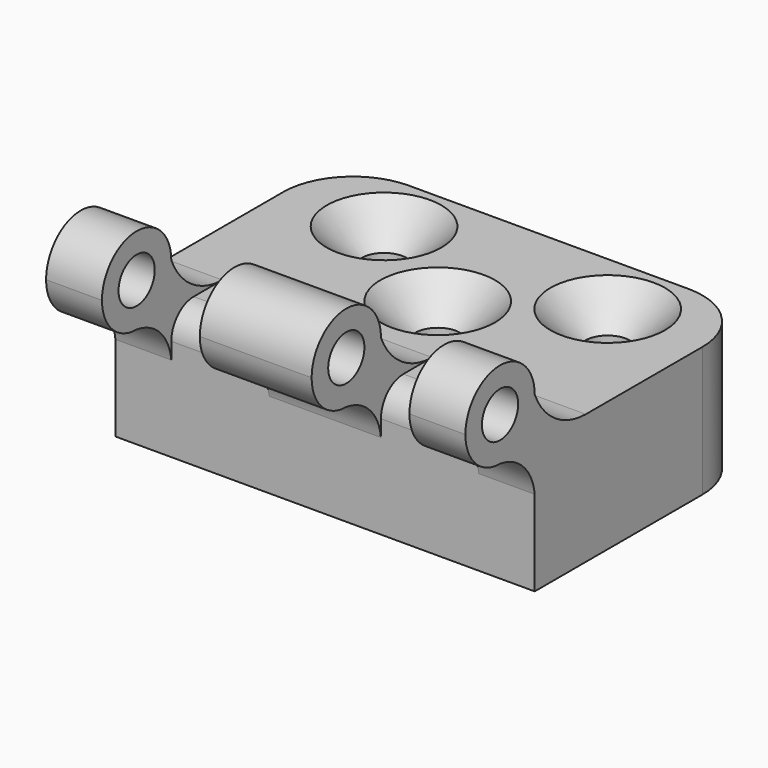
from build123d import *

# Parameters (mm, degrees)
F0_W      = 30
F0_H      = 20
F0_R      = 1.6
F1_DEPTH  = 5
F3_DEPTH  = 30
F7_DEPTH  = 7
F9_DEPTH  = 7
F10_SIZE  = 2.5
F11_R     = 5
F12_R     = 1.6200998357
F13_DEPTH = 30.001
F14_R     = 2
F15_DEPTH = 4.3


with BuildPart() as f1:
    # F0 (on Top) → F1 (new body)
    with BuildSketch(Plane.XY):
        Rectangle(F0_W, F0_H)
        with Locations((-8, 5.2767994255)):
            Circle(F0_R, mode=Mode.SUBTRACT)
        with Locations((0, 0.0767994255)):
            Circle(F0_R, mode=Mode.SUBTRACT)
        with Locations((8, 5.2767994255)):
            Circle(F0_R, mode=Mode.SUBTRACT)
    extrude(amount=F1_DEPTH)

    # F2 (on face) → F3 (join, through all)
    with BuildSketch(Plane(origin=(-15, 0, 0), x_dir=(0, -1, 0), z_dir=(-1, 0, 0))):
        with BuildLine():
            ThreePointArc((13.1, 5), (15.2920310217, 5.9079689783), (16.2, 8.1))
            ThreePointArc((16.2, 8.1), (13.1, 11.2), (10, 8.1))
            ThreePointArc((10, 8.1), (10.9079689783, 5.9079689783), (13.1, 5))
        make_face()
        with BuildLine():
            ThreePointArc((13.1, 5), (10.9079689783, 5.9079689783), (10, 8.1))
            ThreePointArc((10, 8.1), (8.1808280522, 5.8625059643), (5.4291286506, 5))
            Line((5.4291286506, 5), (10, 5))
            Line((10, 5), (10, 1.816622098))
            ThreePointArc((10, 1.816622098), (10.998268655, 3.9455916428), (13.1, 5))
        make_face()
    extrude(amount=-F3_DEPTH)

    # F6 (on offset) → F7 (cut)
    with BuildSketch(Plane.YZ.offset(11)):
        with BuildLine():
            ThreePointArc((-13.1, 5), (-10.9079689783, 5.9079689783), (-10, 8.1))
            ThreePointArc((-10, 8.1), (-15.2920310217, 10.2920310217), (-13.1, 5))
        make_face()
        with BuildLine():
            ThreePointArc((-5.4291286506, 5), (-8.1808280522, 5.8625059643), (-10, 8.1))
            ThreePointArc((-10, 8.1), (-10.9079689783, 5.9079689783), (-13.1, 5))
            ThreePointArc((-13.1, 5), (-10.998268655, 3.9455916428), (-10, 1.816622098))
            Line((-10, 1.816622098), (-10, 5))
            Line((-10, 5), (-5.4291286506, 5))
        make_face()
        with BuildLine():
            Line((-5.3136004135, 5), (-5.4291286506, 5))
            ThreePointArc((-5.4291286506, 5), (-5.371364532, 4.9996666743), (-5.3136004135, 5))
        make_face()
    extrude(amount=-F7_DEPTH, mode=Mode.SUBTRACT)

    # F8 (on offset) → F9 (cut)
    with BuildSketch(Plane(origin=(-11, 0, 0), x_dir=(0, -1, 0), z_dir=(-1, 0, 0))):
        with BuildLine():
            ThreePointArc((13.1, 5), (15.2920310217, 5.9079689783), (16.2, 8.1))
            ThreePointArc((16.2, 8.1), (13.1, 11.2), (10, 8.1))
            ThreePointArc((10, 8.1), (10.9079689783, 5.9079689783), (13.1, 5))
        make_face()
        with BuildLine():
            ThreePointArc((5.3136004135, 5), (5.371364532, 4.9996666743), (5.4291286506, 5))
            Line((5.4291286506, 5), (5.3136004135, 5))
        make_face()
        with BuildLine():
            ThreePointArc((13.1, 5), (10.9079689783, 5.9079689783), (10, 8.1))
            ThreePointArc((10, 8.1), (8.1808280522, 5.8625059643), (5.4291286506, 5))
            Line((5.4291286506, 5), (10, 5))
            Line((10, 5), (10, 1.816622098))
            ThreePointArc((10, 1.816622098), (10.998268655, 3.9455916428), (13.1, 5))
        make_face()
    extrude(amount=-F9_DEPTH, mode=Mode.SUBTRACT)

    # F10
    f10_edges = [f1.edges().sort_by_distance(p)[0] for p in [
        (-9.6, 5.276799, 5),
        (-1.6, 0.076799, 5),
        (6.4, 5.276799, 5),
    ]]
    chamfer(f10_edges, length=F10_SIZE)

    # F11
    f11_edges = [f1.edges().sort_by_distance(p)[0] for p in [
        (-15, 10, 2.5),
        (15, 10, 2.5),
    ]]
    fillet(f11_edges, radius=F11_R)

    # F12 (on face) → F13 (cut, through all)
    with BuildSketch(Plane(origin=(-15, 0, 0), x_dir=(0, -1, 0), z_dir=(-1, 0, 0))):
        with Locations((13.1, 8.1)):
            Circle(F12_R)
    extrude(amount=-F13_DEPTH, mode=Mode.SUBTRACT)

    # F14
    f14_edges = [f1.edges().sort_by_distance(p)[0] for p in [
        (-7.5, -10, 5),
        (7.5, -10, 5),
    ]]
    fillet(f14_edges, radius=F14_R)

    # F15 (add): a face of the model
    f15_faces = [f1.faces().sort_by_distance(p)[0] for p in [
        (14.6394448725, -2.5, 0),
    ]]
    extrude(f15_faces, amount=F15_DEPTH)


solid = f1.part
